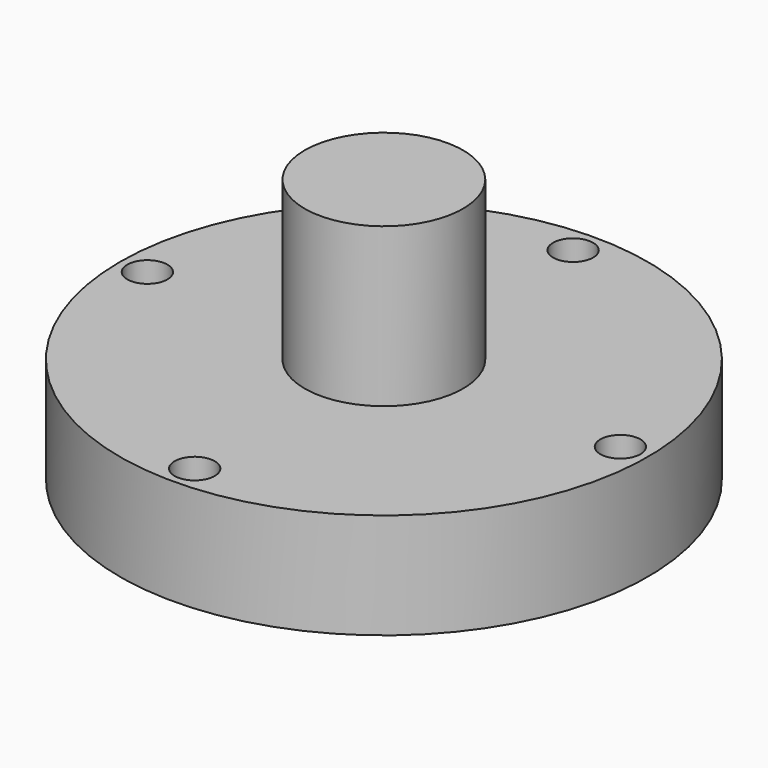
from build123d import *

# Parameters (mm, degrees)
F3_D            = 4.826
F3_COPIES_COUNT = 4


# Not quite as in the source:
# - a pattern or mirror of a feature is missing from the dataset's text; its kind, count and spacing are read off the source's solid


with BuildPart() as f1:
    # F0 (on Front) → F1 (revolve)
    with BuildSketch(Plane.XZ):
        Polygon((-31.75, 0), (0, 0), (0, 31.75), (-9.525, 31.75), (-9.525, 12.7), (-31.75, 12.7), align=None)
    revolve(axis=Axis((0, 0, 15.875), (0, 0, -1)))

    # F3 (through all)
    with Locations(Plane.XY.offset(12.7)):
        with Locations((0, 28.448)):
            f3 = Hole(F3_D / 2)

    # F3_copies: F3 ×4 about axis
    f3_copies_axis = Axis((0, 0, 0), (0, 0, 1))
    for i in range(1, F3_COPIES_COUNT):
        add(f3.rotate(f3_copies_axis, i * 360 / F3_COPIES_COUNT), mode=Mode.SUBTRACT)


solid = f1.part
